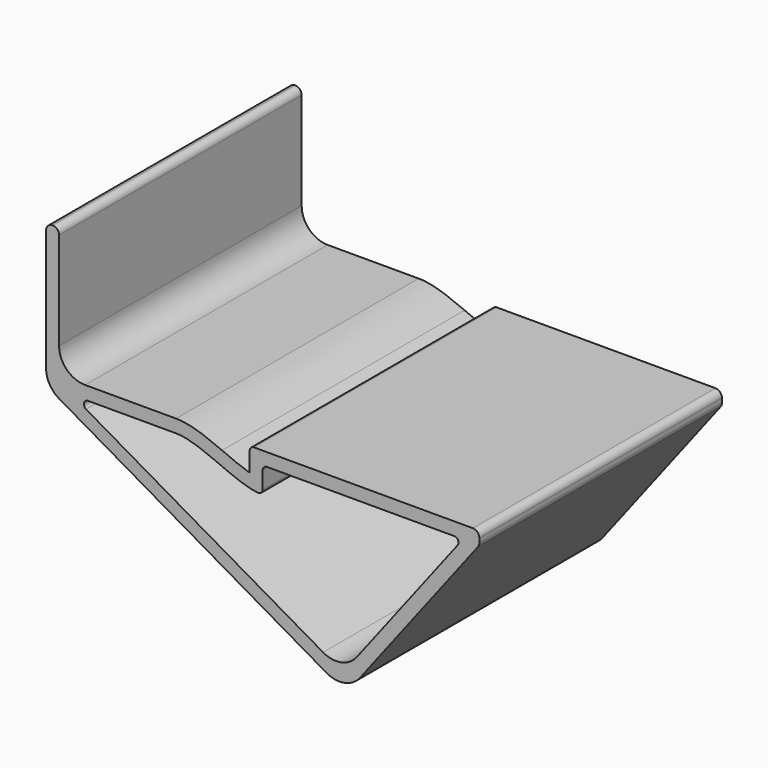
from build123d import *

# Parameters (mm, degrees)
F0_W         = 1.5
F0_H         = 15
F0_H_2       = 1.5
F1_DEPTH     = 35
F2_R         = 3
F3_R         = 0.5
F4_R         = 0.74999
F5_TEXT_SIZE = 7.8123211902
F6_DEPTH     = 0.4


# Not quite as in the source:
# - a fillet or chamfer is up to 0.001 mm smaller than in the source, because OpenCascade refuses the exact size
# - ends of sketch curves that miss each other by under 0.0002 mm in the source are joined
# - Text() gives the source's letters only with a copy of the font that has no kerning and outlines rounded to 1/6400 em; it was checked with that copy


with BuildPart() as f1:
    # F0 (on Front) → F1 (new body)
    with BuildSketch(Plane.XZ):
        with Locations((0.75, 9)):
            Rectangle(F0_W, F0_H)
        with BuildLine():
            Line((1.5, 1.5), (0, 1.5))
            Line((0, 1.5), (0, 0))
            Line((0, 0), (3, 0))
            Line((3, 0), (15, 0))
            Line((15, 0), (20.3076726165, 0))
            add(Edge.make_bspline(
                [(20.3076726165, 0), (19.9613391426, 0.1480763703), (19.1624921639, 0.4865686334), (17.8864112021, 0.9748848409), (16.4769611274, 1.3772161031), (15.5, 1.5), (15, 1.5)],
                knots=[0.5268596167, 0.5268596167, 0.5268596167, 0.5268596167, 0.625, 0.75, 0.875, 1, 1, 1, 1], degree=3))
            Line((15, 1.5), (1.5, 1.5))
        make_face()
        with BuildLine():
            add(Edge.make_bspline(
                [(23.5000271172, -1.2432669014), (23.3597225948, -1.2025116169), (22.8440957766, -1.0410149339), (21.8859439585, -0.6761057841), (20.9362434779, -0.2693177997), (20.4024591259, -0.0405263808), (20.3076726165, 0)],
                knots=[0.2014712136, 0.2014712136, 0.2014712136, 0.2014712136, 0.25, 0.375, 0.5, 0.5268596167, 0.5268596167, 0.5268596167, 0.5268596167], degree=3))
            Line((20.3076726165, 0), (15, 0))
            add(Edge.make_bspline(
                [(25, -3), (22, -3), (18, 0), (15, 0)],
                knots=[0, 0, 0, 0, 10.4403065089, 10.4403065089, 10.4403065089, 10.4403065089], degree=3))
            Line((25, -3), (25, 0))
            Line((25, 0), (23.5, 0))
            Line((23.5, 0), (23.5000271172, -1.2432669014))
        make_face()
        with Locations((24.25, 0.75)):
            Rectangle(F0_W, F0_H_2)
        Polygon((48.1087230729, 0), (50, 0), (50, 1.5), (25, 1.5), (25, 0), align=None)
        Polygon((35.3910161514, -18.7009618943), (34.6410161514, -20), (50, 0), (48.1087230729, 0), (34.2522400908, -18.0434892292), align=None)
        Polygon((3, 0), (0, 0), (34.6410161514, -20), (35.3910161514, -18.7009618943), (34.2522400908, -18.0434892292), align=None)
    extrude(amount=F1_DEPTH)

    # F2
    f2_edges = [f1.edges().sort_by_distance(p)[0] for p in [
        (1.5, -17.5, 1.5),
        (0, -17.5, 0),
        (34.641016, -17.5, -20),
        (34.25224, -17.5, -18.043489),
    ]]
    fillet(f2_edges, radius=F2_R)

    # F3
    f3_edges = [f1.edges().sort_by_distance(p)[0] for p in [
        (48.108723, -17.5, 0),
        (3, -17.5, 0),
        (15, -17.5, 0),
        (23.5, -17.5, 1.5),
        (25, -17.5, 0),
        (25, -17.5, -3),
    ]]
    fillet(f3_edges, radius=F3_R)

    # F4 (radius 0.75 in the source; OpenCascade refuses exactly that, so slightly less here)
    f4_edges = [f1.edges().sort_by_distance(p)[0] for p in [
        (50, -17.5, 0),
        (50, -17.5, 1.5),
        (1.5, -17.5, 16.5),
        (0, -17.5, 16.5),
    ]]
    fillet(f4_edges, radius=F4_R)

    # F5 (on face) → F6 (cut)
    with BuildSketch(Plane(origin=(0, 0, 0), x_dir=(0.8660254038, 0, -0.5), z_dir=(-0.5, 0, -0.8660254038))):
        with Locations((3.5510800735, 14.6875643715)):
            Text('AIRSTER', F5_TEXT_SIZE, font='Open Sans', font_style=FontStyle.BOLD, text_align=(TextAlign.LEFT, TextAlign.BOTTOM))
    extrude(amount=-F6_DEPTH, mode=Mode.SUBTRACT)


solid = f1.part
